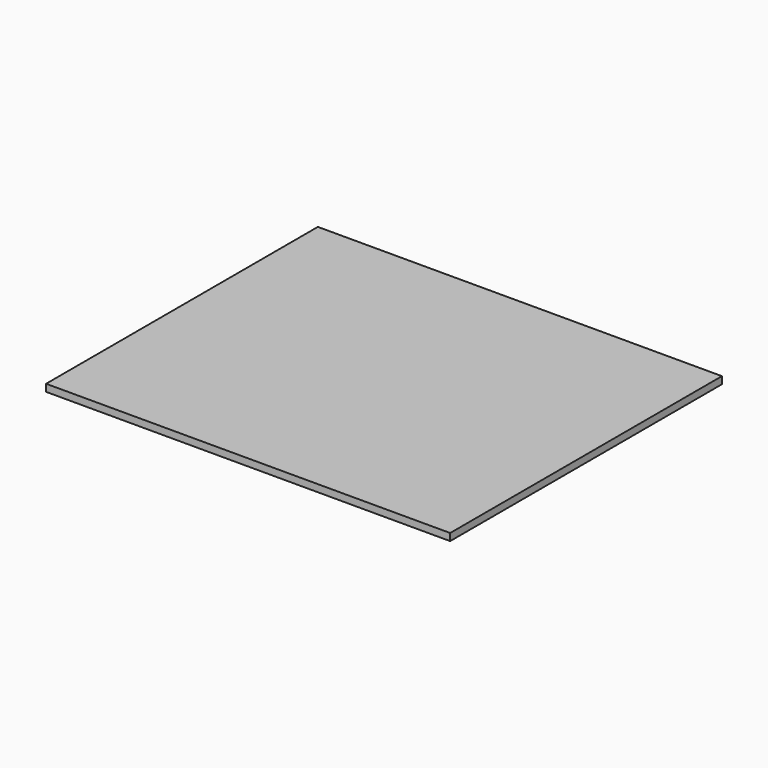
from build123d import *

# Parameters (mm, degrees)
F1_W     = 358.8004
F1_H     = 301.6504
F2_DEPTH = 6.35


# Not quite as in the source:
# - a variable given as a bare number and used for a length is read in inches; the dataset says mm whatever the document's units were


with BuildPart() as f2:
    # F1 (on Top) → F2 (new body)
    with BuildSketch(Plane.XY):
        with Locations((179.4002, -150.8252)):
            Rectangle(F1_W, F1_H)
    extrude(amount=F2_DEPTH)


solid = f2.part
